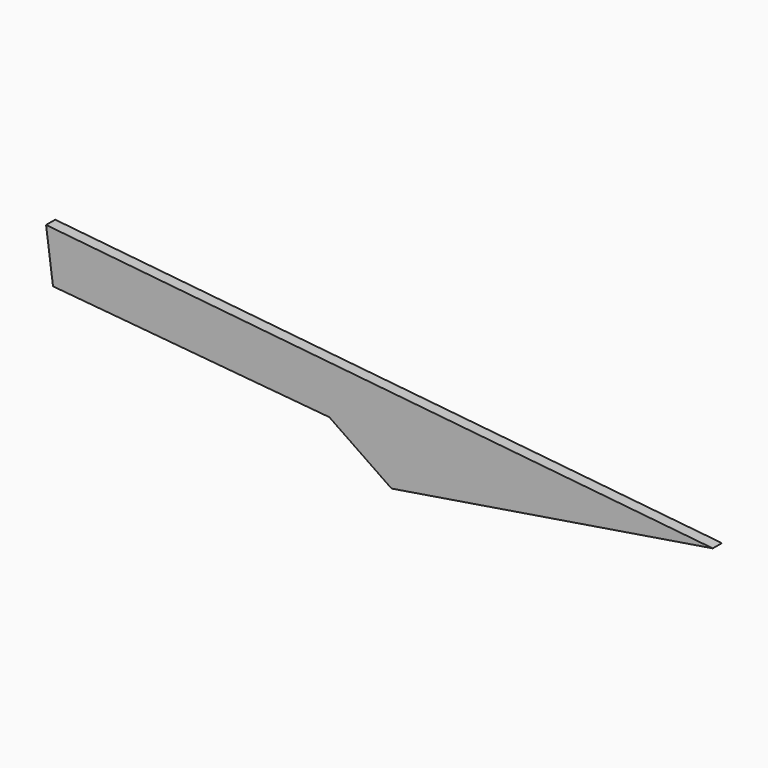
from build123d import *

# Parameters (mm, degrees)
F1_DEPTH = 2.38125


# Not quite as in the source:
# - a length typed as a fraction of an inch, garbled in the dataset ("3 / 203.2 mm" for 3/8 in), is restored


with BuildPart() as f1:
    # F0 (on Front) → F1 (new body)
    with BuildSketch(Plane.XZ):
        Polygon((71.8408152461, 28.3518917859), (-67.275673151, 42.5278358161), (-65.8340528607, 31.7156761885), (-8.1691900268, 26.4297313988), (4.8054051585, 17.5397302955), align=None)
    extrude(amount=F1_DEPTH)


solid = f1.part
